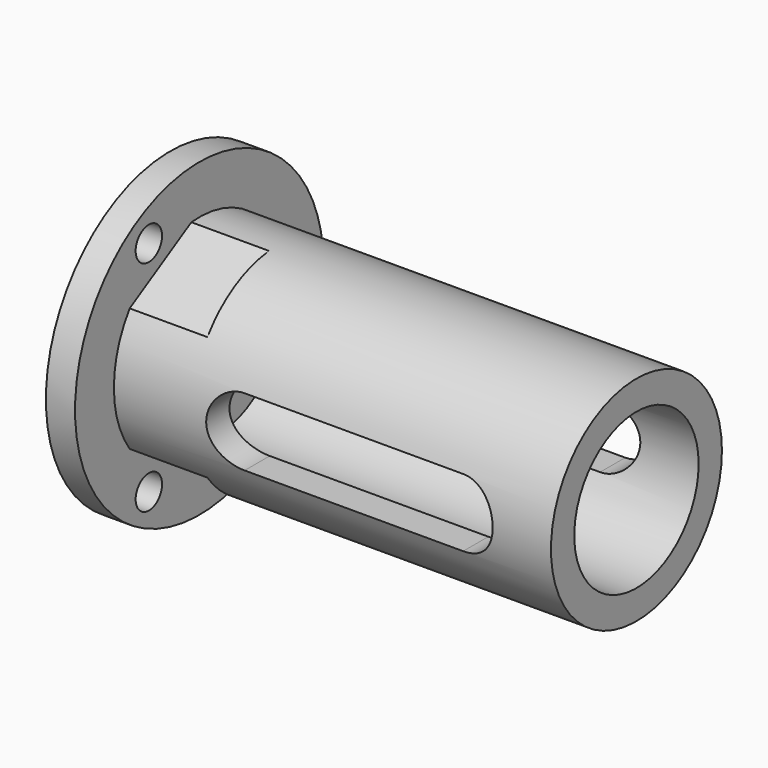
from build123d import *

# Parameters (mm, degrees)
F0_R             = 8
F1_DEPTH         = 1.5
F2_R             = 5.5
F3_DEPTH         = 22.5
F4_R             = 4
F5_DEPTH         = 21.5
F7_D             = 1.7
F9_D             = 3
F11_DEPTH        = 8.001
F11_DEPTH_BACK   = 25
F13_DEPTH        = 4
F13_COPIES_COUNT = 3


# Not quite as in the source:
# - a pattern or mirror of a feature is missing from the dataset's text; its kind, count and spacing are read off the source's solid


with BuildPart() as f1:
    # F0 (on Right) → F1 (new body)
    with BuildSketch(Plane.YZ):
        Circle(F0_R)
    extrude(amount=F1_DEPTH)

    # F2 (on face) → F3 (join)
    with BuildSketch(Plane.YZ.offset(1.5)):
        Circle(F2_R)
    extrude(amount=F3_DEPTH)

    # F4 (on face) → F5 (cut)
    with BuildSketch(Plane.YZ.offset(24)):
        Circle(F4_R)
    extrude(amount=-F5_DEPTH, mode=Mode.SUBTRACT)

    # F7 (through all)
    with Locations(Plane(origin=(0, 0, 0), x_dir=(0, 1, 0), z_dir=(-1, 0, 0))):
        with Locations((-3.25, -5.6291651246), (6.5, 0), (-3.25, 5.6291651246)):
            Hole(F7_D / 2)

    # F9 (through all)
    with Locations(Plane.YZ.offset(2.5)):
        with Locations((0, 0)):
            Hole(F9_D / 2)

    # F10 (on Front) → F11 (cut, two sides)
    with BuildSketch(Plane.XZ) as f11_sk:
        with BuildLine():
            Line((8, -1.75), (19.25, -1.75))
            ThreePointArc((19.25, -1.75), (21, 0), (19.25, 1.75))
            Line((19.25, 1.75), (8, 1.75))
            ThreePointArc((8, 1.75), (6.25, 0), (8, -1.75))
        make_face()
    extrude(amount=-F11_DEPTH, mode=Mode.SUBTRACT)
    extrude(f11_sk.sketch, amount=F11_DEPTH_BACK, mode=Mode.SUBTRACT)

    # F12 (on face) → F13 (cut)
    with BuildSketch(Plane.YZ.offset(1.5)):
        with BuildLine():
            Line((-0.5156865167, -5.4757709427), (-4.4843134833, -3.1844830952))
            ThreePointArc((-4.4843134833, -3.1844830952), (-3.702278018, -4.0673255927), (-2.7500001403, -4.7631396398))
            ThreePointArc((-2.7500001403, -4.7631396398), (-1.6712684341, -5.2399295626), (-0.5156865167, -5.4757709427))
        make_face()
    f13 = extrude(amount=F13_DEPTH, mode=Mode.SUBTRACT)

    # F13_copies: F13 ×3 about axis
    f13_copies_axis = Axis((0, 0, 0), (1, 0, 0))
    for i in range(1, F13_COPIES_COUNT):
        add(f13.rotate(f13_copies_axis, i * 360 / F13_COPIES_COUNT), mode=Mode.SUBTRACT)


solid = f1.part
